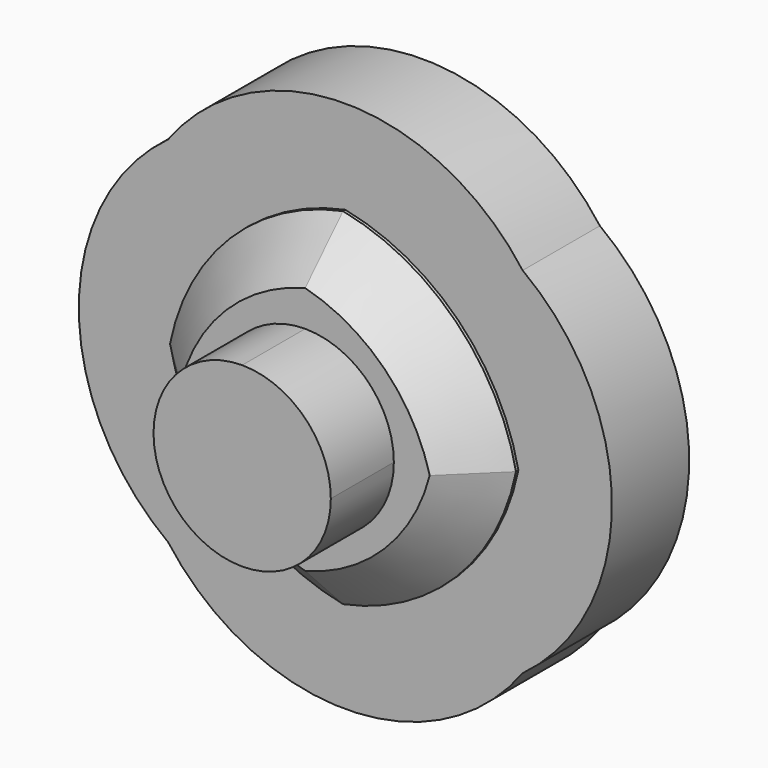
from build123d import *

# Parameters (mm, degrees)
F1_DEPTH = 28.575
F2_DEPTH = 15.875
F3_DEPTH = 7.77875
F4_SIZE  = 7.62


with BuildPart() as f1:
    # F0 (on Front) → F1 (new body, symmetric)
    with BuildSketch(Plane.XZ):
        with BuildLine():
            Line((-14.2875, 0), (0, 0))
            Line((0, 0), (0, 14.2875))
            ThreePointArc((0, 14.2875), (-10.102788, 10.102788), (-14.2875, 0))
        make_face()
        with BuildLine():
            ThreePointArc((-14.2875, 0), (-10.102788, -10.102788), (0, -14.2875))
            Line((0, -14.2875), (0, 0))
            Line((0, 0), (-14.2875, 0))
        make_face()
        with BuildLine():
            Line((0, 0), (0, -14.2875))
            ThreePointArc((0, -14.2875), (10.102788, -10.102788), (14.2875, 0))
            Line((14.2875, 0), (0, 0))
        make_face()
        with BuildLine():
            Line((0, 14.2875), (0, 0))
            Line((0, 0), (14.2875, 0))
            ThreePointArc((14.2875, 0), (10.102788, 10.102788), (0, 14.2875))
        make_face()
    extrude(amount=F1_DEPTH, both=True)

    # F0 (on Front) → F2 (join, symmetric)
    with BuildSketch(Plane.XZ):
        with BuildLine():
            ThreePointArc((0, 27.882225), (-18.159717, 18.159717), (-27.882225, 0))
            Line((-27.882225, 0), (-14.2875, 0))
            ThreePointArc((-14.2875, 0), (-10.102788, 10.102788), (0, 14.2875))
            Line((0, 14.2875), (0, 27.882225))
        make_face()
        with BuildLine():
            Line((14.2875, 0), (27.882225, 0))
            ThreePointArc((27.882225, 0), (18.159717, 18.159717), (0, 27.882225))
            Line((0, 27.882225), (0, 14.2875))
            ThreePointArc((0, 14.2875), (10.102788, 10.102788), (14.2875, 0))
        make_face()
        with BuildLine():
            Line((0, -14.2875), (0, -27.882225))
            ThreePointArc((0, -27.882225), (18.159717, -18.159717), (27.882225, 0))
            Line((27.882225, 0), (14.2875, 0))
            ThreePointArc((14.2875, 0), (10.102788, -10.102788), (0, -14.2875))
        make_face()
        with BuildLine():
            ThreePointArc((-27.882225, 0), (-18.159717, -18.159717), (0, -27.882225))
            Line((0, -27.882225), (0, -14.2875))
            ThreePointArc((0, -14.2875), (-10.102788, -10.102788), (-14.2875, 0))
            Line((-14.2875, 0), (-27.882225, 0))
        make_face()
    extrude(amount=F2_DEPTH, both=True)

    # F0 (on Front) → F3 (join, symmetric)
    with BuildSketch(Plane.XZ):
        with BuildLine():
            ThreePointArc((28.575, 28.575), (0, 42.969392), (-28.575, 28.575))
            ThreePointArc((-28.575, 28.575), (-42.969392, 0), (-28.575, -28.575))
            ThreePointArc((-28.575, -28.575), (0, -42.969392), (28.575, -28.575))
            ThreePointArc((28.575, -28.575), (42.969392, 0), (28.575, 28.575))
        make_face()
        with BuildLine():
            ThreePointArc((27.882225, 0), (18.159717, -18.159717), (0, -27.882225))
            ThreePointArc((0, -27.882225), (-18.159717, -18.159717), (-27.882225, 0))
            ThreePointArc((-27.882225, 0), (-18.159717, 18.159717), (0, 27.882225))
            ThreePointArc((0, 27.882225), (18.159717, 18.159717), (27.882225, 0))
        make_face(mode=Mode.SUBTRACT)
    extrude(amount=F3_DEPTH, both=True)

    # F4
    f4_edges = [f1.edges().sort_by_distance(p)[0] for p in [
        (-18.159717, -15.875, -18.159717),
        (-18.159717, -15.875, 18.159717),
        (18.159717, -15.875, -18.159717),
        (18.159717, -15.875, 18.159717),
        (-18.159717, 15.875, 18.159717),
        (-18.159717, 15.875, -18.159717),
        (18.159717, 15.875, -18.159717),
        (18.159717, 15.875, 18.159717),
    ]]
    chamfer(f4_edges, length=F4_SIZE)


solid = f1.part
